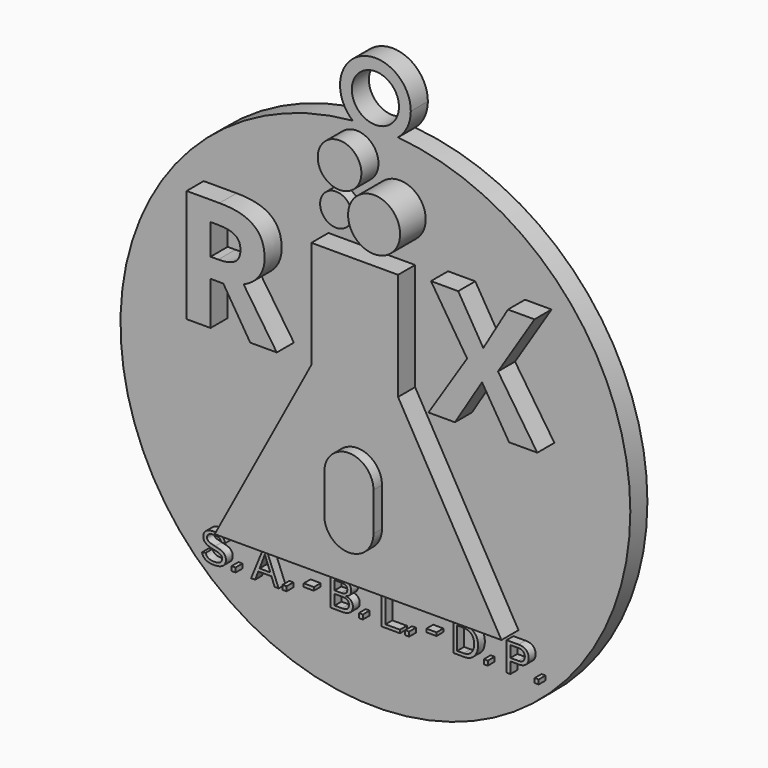
from build123d import *

# Parameters (mm, degrees)
F3_DEPTH      = 5.08
F4_DEPTH      = 6.35
F2_TEXT_SIZE  = 48.5385936271
F5_DEPTH      = 6.35
F7_TEXT_SIZE  = 47.0373986496
F8_DEPTH      = 6.35
F10_R         = 7.740834859
F11_DEPTH     = 9.525
F9_R          = 6.4951543257
F13_DEPTH     = 6.35
F12_R         = 4.7467233393
F14_DEPTH     = 3.175
F15_TEXT_SIZE = 12.3871754329
F16_DEPTH     = 2.54
F6_W          = 14.6283619106
F6_H          = 11.4489616826
F17_DEPTH     = 3.175
F0_R          = 7.009301185
F18_DEPTH     = 6.35


# Not quite as in the source:
# - Text() gives the source's letters only with a copy of the font that has no kerning and outlines rounded to 1/6400 em; it was checked with that copy


with BuildPart() as f3:
    # F0 (on Front) → F3 (new body)
    with BuildSketch(Plane.XZ):
        with BuildLine():
            ThreePointArc((-6.7387393639, 75.5405327853), (0, 73.1007905486), (6.7387393639, 75.5405327853))
            ThreePointArc((6.7387393639, 75.5405327853), (0, 75.8405083165), (-6.7387393639, 75.5405327853))
        make_face()
        with BuildLine():
            ThreePointArc((-6.7387393639, 75.5405327853), (-51.1894192335, -55.9591463501), (75.8405083165, 0))
            ThreePointArc((75.8405083165, 0), (55.9591463501, 51.1894192335), (6.7387393639, 75.5405327853))
            ThreePointArc((6.7387393639, 75.5405327853), (0, 73.1007905486), (-6.7387393639, 75.5405327853))
        make_face()
    extrude(amount=-F3_DEPTH)

    # F1 (on face) → F4 (join)
    with BuildSketch(Plane.XZ):
        Polygon((11.8166133761, 43.774805963), (-13.9767182991, 43.774805963), (-13.9767182991, 11.7799239233), (-42.7191470753, -41.8699160218), (42.574994266, -41.8699160218), (11.8166133761, 11.7799239233), align=None)
    extrude(amount=F4_DEPTH)

    # F2 (on face) → F5 (join)
    with BuildSketch(Plane.XZ):
        with Locations((20.8709221333, 10.6643661857)):
            Text('X', F2_TEXT_SIZE, font='Open Sans', font_style=FontStyle.BOLD, text_align=(TextAlign.LEFT, TextAlign.BOTTOM))
    extrude(amount=F5_DEPTH)

    # F7 (on face) → F8 (join)
    with BuildSketch(Plane.XZ):
        with Locations((-55.3039684892, 11.7093101144)):
            Text('R', F7_TEXT_SIZE, font='Open Sans', font_style=FontStyle.BOLD, text_align=(TextAlign.LEFT, TextAlign.BOTTOM))
    extrude(amount=F8_DEPTH)

    # F10 (on face) → F11 (join)
    with BuildSketch(Plane.XZ):
        with Locations((7.2273598053, 56.7394308746)):
            Circle(F10_R)
    extrude(amount=F11_DEPTH)

    # F9 (on face) → F13 (join)
    with BuildSketch(Plane.XZ):
        with Locations((-5.5844392627, 66.8331310153)):
            Circle(F9_R)
    extrude(amount=F13_DEPTH)

    # F12 (on face) → F14 (join)
    with BuildSketch(Plane.XZ):
        with Locations((-9.1603510082, 52.7318492532)):
            Circle(F12_R)
    extrude(amount=F14_DEPTH)

    # F15 (on face) → F16 (join)
    with BuildSketch(Plane.XZ):
        with Locations((-50.1337179526, -52.4541754917)):
            Text('S. A. - B. L. - D. P.', F15_TEXT_SIZE, font='Arimo', text_align=(TextAlign.LEFT, TextAlign.BOTTOM))
    extrude(amount=F16_DEPTH)

    # F6 (on face) → F17 (join)
    with BuildSketch(Plane.XZ.offset(6.35)):
        with BuildLine():
            Line((7.0389551111, -24.2859181017), (-7.5894067995, -24.2859181017))
            ThreePointArc((-7.5894067995, -24.2859181017), (-0.2752258442, -31.600099057), (7.0389551111, -24.2859181017))
        make_face()
        with Locations((-0.2752258442, -18.5614372604)):
            Rectangle(F6_W, F6_H)
        with BuildLine():
            ThreePointArc((7.0389551111, -12.8369564191), (-0.2752258442, -5.5227754638), (-7.5894067995, -12.8369564191))
            Line((-7.5894067995, -12.8369564191), (7.0389551111, -12.8369564191))
        make_face()
    extrude(amount=F17_DEPTH)

    # F0 (on Front) → F18 (join)
    with BuildSketch(Plane.XZ):
        with BuildLine():
            ThreePointArc((-6.7387393639, 75.5405327853), (-51.1894192335, -55.9591463501), (75.8405083165, 0))
            ThreePointArc((75.8405083165, 0), (55.9591463501, 51.1894192335), (6.7387393639, 75.5405327853))
            ThreePointArc((6.7387393639, 75.5405327853), (0, 73.1007905486), (-6.7387393639, 75.5405327853))
        make_face()
        with BuildLine():
            ThreePointArc((-6.7387393639, 75.5405327853), (0, 73.1007905486), (6.7387393639, 75.5405327853))
            ThreePointArc((6.7387393639, 75.5405327853), (0, 75.8405083165), (-6.7387393639, 75.5405327853))
        make_face()
        with BuildLine():
            ThreePointArc((-6.7387393639, 75.5405327853), (0, 75.8405083165), (6.7387393639, 75.5405327853))
            ThreePointArc((6.7387393639, 75.5405327853), (9.5325015533, 79.1622850906), (10.52630676, 83.6270973086))
            ThreePointArc((10.52630676, 83.6270973086), (-4.4648122181, 93.1595988619), (-6.7387393639, 75.5405327853))
        make_face()
        with Locations((0, 83.6270973086)):
            Circle(F0_R, mode=Mode.SUBTRACT)
    extrude(amount=-F18_DEPTH)


solid = f3.part
